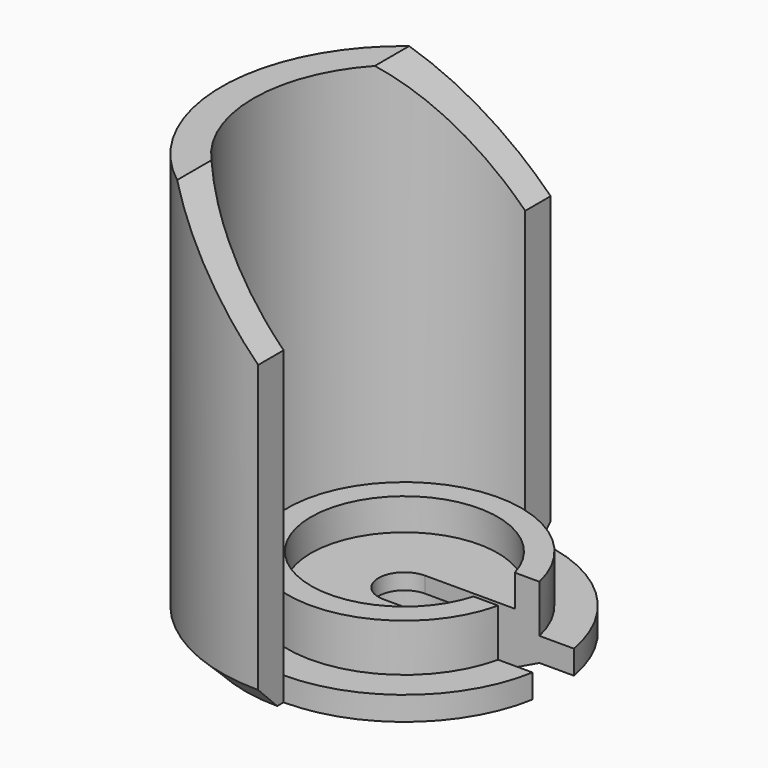
from build123d import *

# Parameters (mm, degrees)
F1_DEPTH    = 3
F2_DEPTH    = 1
F3_DEPTH    = 3.5
F4_DEPTH    = 1.5
F5_DEPTH    = 1.5
F6_DEPTH    = 25
F7_T1_DEPTH = 38.0035618315
F7_T3_DEPTH = 38.0035618315
F8_SIZE2    = 3.99999
F8_SIZE     = 1.99999
F9_SIZE     = 1.5


# Not quite as in the source:
# - a fillet or chamfer that OpenCascade refuses, or shapes differently, is made with other operations: its cross-section is extruded or revolved along the edge and cut away or added
# - a fillet or chamfer is up to 0.001 mm smaller than in the source, because OpenCascade refuses the exact size


with BuildPart() as f1:
    # F0 (on Top) → F1 (new body)
    with BuildSketch(Plane.XY):
        with BuildLine():
            Line((5.6457948953, 1.625), (7.193747285, 1.625))
            ThreePointArc((7.193747285, 1.625), (-7.375, 0), (7.193747285, -1.625))
            Line((7.193747285, -1.625), (5.6457948953, -1.625))
            ThreePointArc((5.6457948953, -1.625), (-5.875, 0), (5.6457948953, 1.625))
        make_face()
    extrude(amount=F1_DEPTH)

    # F0 (on Top) → F2 (join)
    with BuildSketch(Plane.XY):
        with BuildLine():
            Line((2.3717082451, 1.625), (5.6457948953, 1.625))
            ThreePointArc((5.6457948953, 1.625), (-5.875, 0), (5.6457948953, -1.625))
            Line((5.6457948953, -1.625), (2.3717082451, -1.625))
            ThreePointArc((2.3717082451, -1.625), (-2.875, 0), (2.3717082451, 1.625))
        make_face()
        with BuildLine():
            Line((0, 1.625), (2.3717082451, 1.625))
            ThreePointArc((2.3717082451, 1.625), (-2.875, 0), (2.3717082451, -1.625))
            Line((2.3717082451, -1.625), (0, -1.625))
            ThreePointArc((0, -1.625), (-1.625, 0), (0, 1.625))
        make_face()
    extrude(amount=F2_DEPTH)

    # F0 (on Top) → F3 (join)
    with BuildSketch(Plane.XY):
        with BuildLine():
            Line((5.6457948953, 1.625), (7.193747285, 1.625))
            ThreePointArc((7.193747285, 1.625), (-7.375, 0), (7.193747285, -1.625))
            Line((7.193747285, -1.625), (5.6457948953, -1.625))
            ThreePointArc((5.6457948953, -1.625), (-5.875, 0), (5.6457948953, 1.625))
        make_face()
        with BuildLine():
            Line((2.3717082451, 1.625), (5.6457948953, 1.625))
            ThreePointArc((5.6457948953, 1.625), (-5.875, 0), (5.6457948953, -1.625))
            Line((5.6457948953, -1.625), (2.3717082451, -1.625))
            ThreePointArc((2.3717082451, -1.625), (-2.875, 0), (2.3717082451, 1.625))
        make_face()
    extrude(amount=-F3_DEPTH)

    # F0 (on Top) → F4 (join)
    with BuildSketch(Plane.XY):
        with BuildLine():
            Line((7.193747285, 1.625), (9.3599879808, 1.625))
            ThreePointArc((9.3599879808, 1.625), (6.1160649114, 7.2693706743), (0, 9.5))
            ThreePointArc((0, 9.5), (-9.5, 0), (0, -9.5))
            ThreePointArc((0, -9.5), (6.1160649114, -7.2693706743), (9.3599879808, -1.625))
            Line((9.3599879808, -1.625), (7.193747285, -1.625))
            ThreePointArc((7.193747285, -1.625), (-7.375, 0), (7.193747285, 1.625))
        make_face()
    extrude(amount=-F4_DEPTH)

    # F0 (on Top) → F5 (join)
    with BuildSketch(Plane.XY):
        with BuildLine():
            ThreePointArc((0, -9.5), (-9.5, 0), (0, 9.5))
            Line((0, 9.5), (0, 11.5))
            ThreePointArc((0, 11.5), (-11.5, 0), (0, -11.5))
            Line((0, -11.5), (0, -9.5))
        make_face()
    extrude(amount=-F5_DEPTH)

    # F0 (on Top) → F6 (join)
    with BuildSketch(Plane.XY):
        with BuildLine():
            ThreePointArc((0, -9.5), (-9.5, 0), (0, 9.5))
            Line((0, 9.5), (0, 11.5))
            ThreePointArc((0, 11.5), (-11.5, 0), (0, -11.5))
            Line((0, -11.5), (0, -9.5))
        make_face()
    extrude(amount=F6_DEPTH)

    # F7: chamfer of 7 on 2 edges, made by hand

    # F7_s2 → F7_t1 (cut)
    with BuildSketch(Plane.XZ.offset(-8.5017809158)):
        Polygon((-7, 25), (0, 18), (0, 25), align=None)
    extrude(amount=F7_T1_DEPTH, mode=Mode.SUBTRACT)

    # F7_s4 → F7_t3 (cut)
    with BuildSketch(Plane.XZ.offset(-29.5017809158)):
        Polygon((0, 18), (-7, 25), (0, 25), align=None)
    extrude(amount=F7_T3_DEPTH, mode=Mode.SUBTRACT)

    # F8 (size 2 and 4 in the source; OpenCascade refuses exactly that, so slightly less here)
    f8_edges = [f1.edges().sort_by_distance(p)[0] for p in [
        (-7.375, 0, -3.5),
    ]]
    f8_side = f1.faces().sort_by_distance((-7.375, 0, -2.5))[0]
    chamfer(f8_edges, length=F8_SIZE, length2=F8_SIZE2, reference=f8_side)

    # F9
    f9_edges = [f1.edges().sort_by_distance(p)[0] for p in [
        (-11.5, 0, -1.5),
    ]]
    chamfer(f9_edges, length=F9_SIZE)


solid = f1.part
